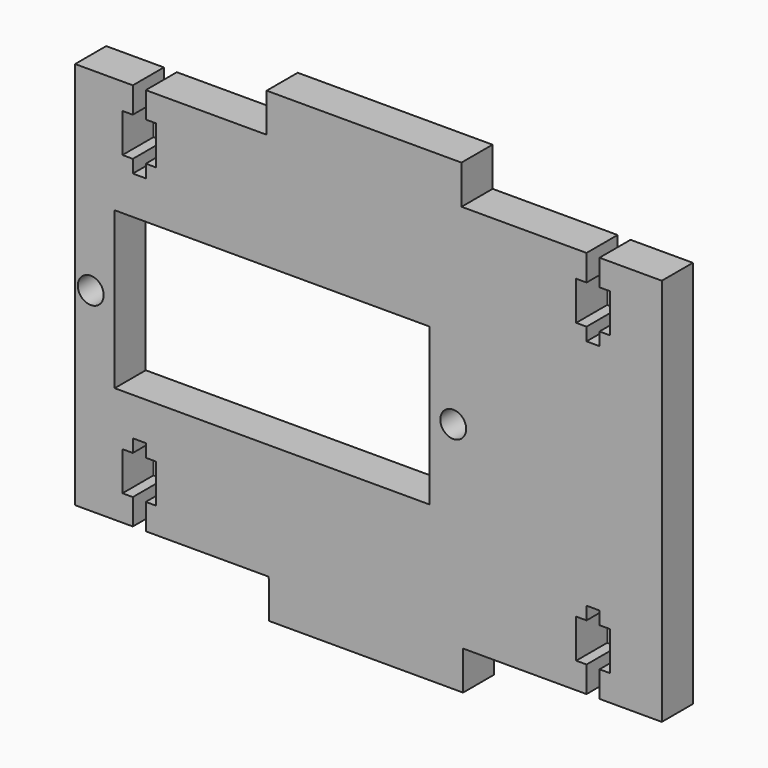
from build123d import *

# Parameters (mm, degrees)
F3_W     = 24.3006017764
F3_H     = 12.100000065
F3_R     = 1
F4_DEPTH = 3


# Not quite as in the source:
# - ends of sketch curves that miss each other by under 0.0002 mm in the source are joined


with BuildPart() as f4:
    # F3 (on Front) → F4 (new body)
    with BuildSketch(Plane.XZ):
        Polygon((-18.3427034128, 0), (-17.3427034128, 0), (-17.3423305717, 1.9999998262), (-18.1417713099, 1.9999998262), (-18.1417713099, 4.9999998262), (-17.3417713099, 4.9999998262), (-17.3415848893, 5.9999998262), (-16.3415848684, 5.9999998262), (-16.3417712925, 4.9999998262), (-15.5417712925, 4.9999998262), (-15.5417712925, 1.9999998262), (-16.3423305647, 1.9999998262), (-16.3427034128, 0), (-15.3427034128, 0), (-6.8427034128, 0), (8.1310835591, 0), (8.1572965872, 0), (16.6572965872, 0), (17.7038592511, 0), (17.704234553, 2.0131421474), (16.9047938148, 2.0131421517), (16.9047938308, 5.0131421517), (17.7047938308, 5.0131421474), (17.7049802567, 6.0131421474), (18.7049802776, 6.0131421421), (18.7047938482, 5.0131421421), (19.5047938482, 5.0131421378), (19.5047938321, 2.0131421378), (18.7042345599, 2.0131421421), (18.703859251, 0), (19.6572965872, 0), (23.5180836171, 0), (23.5180836171, 30), (18.7038593313, 30), (18.7042346294, 27.9868579887), (19.5047939016, 27.9868579887), (19.5047939016, 24.9868579887), (18.7047939016, 24.9868579887), (18.7049803257, 23.9868579887), (17.7049803048, 23.9868579887), (17.7047938842, 24.9868579887), (16.9047938842, 24.9868579887), (16.9047938842, 27.9868579887), (17.7042346225, 27.9868579887), (17.7038593313, 30), (8.0515714362, 30), (0, 30), (-7.0037143305, 30), (-16.3427034128, 30), (-16.3423305647, 28.0000001738), (-15.5417712925, 28.0000001738), (-15.5417712925, 25.0000001738), (-16.3417712925, 25.0000001738), (-16.3415848684, 24.0000001738), (-17.3415848893, 24.0000001738), (-17.3417713099, 25.0000001738), (-18.1417713099, 25.0000001738), (-18.1417713099, 28.0000001738), (-17.3423305717, 28.0000001738), (-17.3427034128, 30), (-21.7979144805, 30), (-21.7979144805, 28.0000001738), (-21.7979144805, 25.0000001738), (-21.7979144805, 24.0000001738), (-21.7979144805, 15.0000001738), (-21.7979144805, 1.738e-07), align=None)
        with BuildLine():
            ThreePointArc((-19.593004301, 15.0000001705), (-20.5930043024, 14.0000001705), (-21.593004301, 15.0000001732))
            ThreePointArc((-21.593004301, 15.0000001732), (-20.5930042997, 16.0000001705), (-19.593004301, 15.0000001705))
        make_face(mode=Mode.SUBTRACT)
        with Locations((-6.593004301, 15.0000001331)):
            Rectangle(F3_W, F3_H, mode=Mode.SUBTRACT)
        with Locations((7.406995699, 15.0000000956)):
            Circle(F3_R, mode=Mode.SUBTRACT)
        Polygon((-7.0037143305, 33), (-7.0037143305, 30), (0, 30), (8.0515714362, 30), (8.0409989211, 33), align=None)
        Polygon((8.1310835591, 0), (-6.8427034128, 0), (-6.826602321, -3), (0, -3), (8.1678691023, -3), (8.1572965872, 0), align=None)
    extrude(amount=F4_DEPTH)


solid = f4.part
